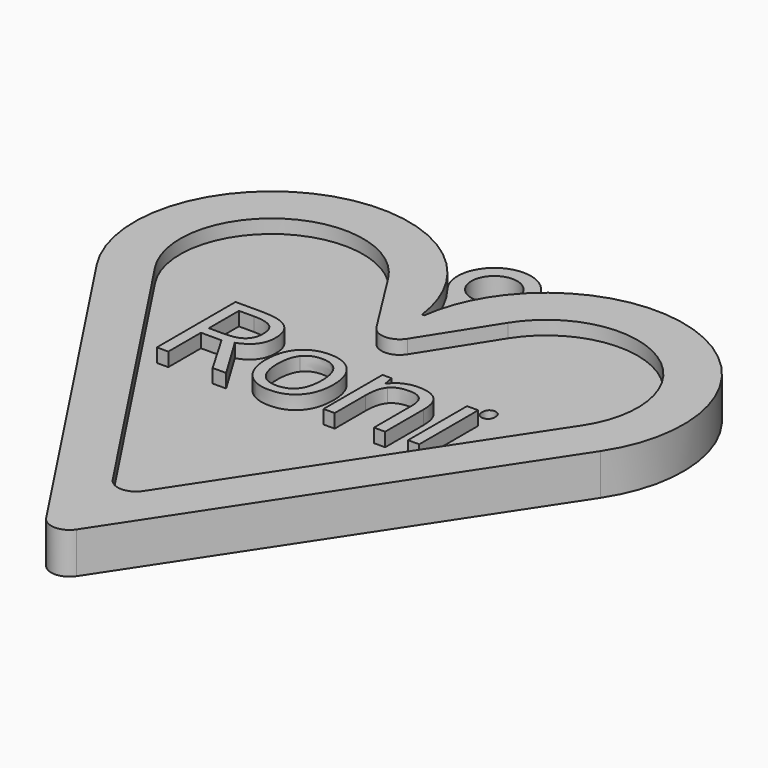
from build123d import *

# Parameters (mm, degrees)
F0_W     = 1.2206887795
F0_H     = 8.0556051444
F0_R     = 2.5
F1_DEPTH = 3
F2_DEPTH = 4.5
F3_R     = 2


# Not quite as in the source:
# - a feature names something its author has since deleted; it is built from what else it names


with BuildPart() as f1:
    # F0 (on Top) → F1 (new body)
    with BuildSketch(Plane.XY):
        with BuildLine():
            Line((-36.7494719235, 22.4924636665), (-36.8790277196, 22.5606875716))
            ThreePointArc((-36.8790277196, 22.5606875716), (-37.9113762546, 26.3820166599), (-39.9073666892, 29.800250368))
            ThreePointArc((-39.9073666892, 29.800250368), (-60.4879285093, 32.7852591337), (-64.2724077033, 12.336603447))
            Line((-64.2724077033, 12.336603447), (-36.7494719235, -29.406515819))
            Line((-36.7494719235, -29.406515819), (-9.2265361436, 12.336603447))
            ThreePointArc((-9.2265361436, 12.336603447), (-13.0110153192, 32.7852591205), (-33.5915771299, 29.8002504037))
            ThreePointArc((-33.5915771299, 29.8002504037), (-35.5875675836, 26.3820166807), (-36.6199161273, 22.5606875716))
            Line((-36.6199161273, 22.5606875716), (-36.7494719235, 22.4924636665))
        make_face()
        with BuildLine():
            Line((-36.7494719235, -20.3231824857), (-60.0980957767, 15.088897025))
            ThreePointArc((-60.0980957767, 15.088897025), (-57.1762344668, 28.9929037025), (-43.2999821807, 25.9419534093))
            Line((-43.2999821807, 25.9419534093), (-36.7494719235, 15.593484181))
            Line((-36.7494719235, 15.593484181), (-30.1989616662, 25.9419534093))
            ThreePointArc((-30.1989616662, 25.9419534093), (-16.3227093801, 28.9929037025), (-13.4008480702, 15.088897025))
            Line((-13.4008480702, 15.088897025), (-36.7494719235, -20.3231824857))
        make_face(mode=Mode.SUBTRACT)
        with BuildLine():
            ThreePointArc((-43.2999821807, 25.9419534093), (-57.1762344668, 28.9929037025), (-60.0980957767, 15.088897025))
            Line((-60.0980957767, 15.088897025), (-36.7494719235, -20.3231824857))
            Line((-36.7494719235, -20.3231824857), (-13.4008480702, 15.088897025))
            ThreePointArc((-13.4008480702, 15.088897025), (-16.3227093801, 28.9929037025), (-30.1989616662, 25.9419534093))
            Line((-30.1989616662, 25.9419534093), (-36.7494719235, 15.593484181))
            Line((-36.7494719235, 15.593484181), (-43.2999821807, 25.9419534093))
        make_face()
        with BuildLine():
            Line((-47.2641347396, 8.1347208725), (-49.5079441725, 8.1347208725))
            Line((-49.5079441725, 8.1347208725), (-49.5079441725, 3.6659180187))
            Line((-49.5079441725, 3.6659180187), (-50.7568569701, 3.6659180187))
            Line((-50.7568569701, 3.6659180187), (-50.7568569701, 14.4122128813))
            Line((-50.7568569701, 14.4122128813), (-47.8097990881, 14.4122128813))
            add(Edge.make_bspline(
                [(-47.8097990881, 14.4122128813), (-45.8317658249, 14.4122128813), (-44.8874372219, 13.6548683977)],
                knots=[0, 0, 0, 1, 1, 1], degree=2))
            add(Edge.make_bspline(
                [(-44.8874372219, 13.6548683977), (-43.9431086188, 12.897523914), (-43.9431086188, 11.3757789422)],
                knots=[0, 0, 0, 1, 1, 1], degree=2))
            add(Edge.make_bspline(
                [(-43.9431086188, 11.3757789422), (-43.9431086188, 9.2448655814), (-46.1045979991, 8.4945771023)],
                knots=[0, 0, 0, 1, 1, 1], degree=2))
            Line((-46.1045979991, 8.4945771023), (-43.1857641352, 3.6659180187))
            Line((-43.1857641352, 3.6659180187), (-44.6628210784, 3.6659180187))
            Line((-44.6628210784, 3.6659180187), (-47.2641347396, 8.1347208725))
        make_face(mode=Mode.SUBTRACT)
        with BuildLine():
            add(Edge.make_bspline(
                [(-35.6793513415, 10.7442665389), (-34.6832787054, 9.6188338202), (-34.6832787054, 7.7019525961)],
                knots=[0, 0, 0, 1, 1, 1], degree=2))
            add(Edge.make_bspline(
                [(-34.6832787054, 7.7019525961), (-34.6832787054, 5.7309753374), (-35.6746473385, 4.6243586307)],
                knots=[0, 0, 0, 1, 1, 1], degree=2))
            add(Edge.make_bspline(
                [(-35.6746473385, 4.6243586307), (-36.6660159716, 3.517741924), (-38.4159050891, 3.517741924)],
                knots=[0, 0, 0, 1, 1, 1], degree=2))
            add(Edge.make_bspline(
                [(-38.4159050891, 3.517741924), (-39.49782578, 3.517741924), (-40.3351383147, 4.0257742485)],
                knots=[0, 0, 0, 1, 1, 1], degree=2))
            add(Edge.make_bspline(
                [(-40.3351383147, 4.0257742485), (-41.1724508494, 4.5338065729), (-41.6287391408, 5.4816631782)],
                knots=[0, 0, 0, 1, 1, 1], degree=2))
            add(Edge.make_bspline(
                [(-41.6287391408, 5.4816631782), (-42.0850274322, 6.4295197835), (-42.0850274322, 7.7019525961)],
                knots=[0, 0, 0, 1, 1, 1], degree=2))
            add(Edge.make_bspline(
                [(-42.0850274322, 7.7019525961), (-42.0850274322, 9.6705778533), (-41.0995388029, 10.7701385555)],
                knots=[0, 0, 0, 1, 1, 1], degree=2))
            add(Edge.make_bspline(
                [(-41.0995388029, 10.7701385555), (-40.1140501735, 11.8696992577), (-38.3641610561, 11.8696992577)],
                knots=[0, 0, 0, 1, 1, 1], degree=2))
            add(Edge.make_bspline(
                [(-38.3641610561, 11.8696992577), (-36.6754239776, 11.8696992577), (-35.6793513415, 10.7442665389)],
                knots=[0, 0, 0, 1, 1, 1], degree=2))
        make_face(mode=Mode.SUBTRACT)
        with BuildLine():
            Line((-25.8091770384, 3.6659180187), (-27.0298658179, 3.6659180187))
            Line((-27.0298658179, 3.6659180187), (-27.0298658179, 8.8779533471))
            add(Edge.make_bspline(
                [(-27.0298658179, 8.8779533471), (-27.0298658179, 9.8610899749), (-27.477922104, 10.3467782851)],
                knots=[0, 0, 0, 1, 1, 1], degree=2))
            add(Edge.make_bspline(
                [(-27.477922104, 10.3467782851), (-27.9259783902, 10.8324665953), (-28.8832430015, 10.8324665953)],
                knots=[0, 0, 0, 1, 1, 1], degree=2))
            add(Edge.make_bspline(
                [(-28.8832430015, 10.8324665953), (-30.146267808, 10.8324665953), (-30.7342681836, 10.1492101589)],
                knots=[0, 0, 0, 1, 1, 1], degree=2))
            add(Edge.make_bspline(
                [(-30.7342681836, 10.1492101589), (-31.3222685591, 9.4659537226), (-31.3222685591, 7.8924647178)],
                knots=[0, 0, 0, 1, 1, 1], degree=2))
            Line((-31.3222685591, 7.8924647178), (-31.3222685591, 3.6659180187))
            Line((-31.3222685591, 3.6659180187), (-32.5429573386, 3.6659180187))
            Line((-32.5429573386, 3.6659180187), (-32.5429573386, 11.721523163))
            Line((-32.5429573386, 11.721523163), (-31.5504127047, 11.721523163))
            Line((-31.5504127047, 11.721523163), (-31.3528445786, 10.6184344586))
            Line((-31.3528445786, 10.6184344586), (-31.294044541, 10.6184344586))
            add(Edge.make_bspline(
                [(-31.294044541, 10.6184344586), (-30.9177243007, 11.2134908386), (-30.2415238689, 11.5415950481)],
                knots=[0, 0, 0, 1, 1, 1], degree=2))
            add(Edge.make_bspline(
                [(-30.2415238689, 11.5415950481), (-29.5653234371, 11.8696992577), (-28.7350669068, 11.8696992577)],
                knots=[0, 0, 0, 1, 1, 1], degree=2))
            add(Edge.make_bspline(
                [(-28.7350669068, 11.8696992577), (-27.2791779771, 11.8696992577), (-26.5441775077, 11.1676268093)],
                knots=[0, 0, 0, 1, 1, 1], degree=2))
            add(Edge.make_bspline(
                [(-26.5441775077, 11.1676268093), (-25.8091770384, 10.465554361), (-25.8091770384, 8.9202893741)],
                knots=[0, 0, 0, 1, 1, 1], degree=2))
            Line((-25.8091770384, 8.9202893741), (-25.8091770384, 3.6659180187))
        make_face(mode=Mode.SUBTRACT)
        with Locations((-22.693951049, 7.6937205909)):
            Rectangle(F0_W, F0_H, mode=Mode.SUBTRACT)
        with BuildLine():
            add(Edge.make_bspline(
                [(-23.2019833734, 13.2903081649), (-23.4077835048, 13.492580294), (-23.4077835048, 13.9041805569)],
                knots=[0, 0, 0, 1, 1, 1], degree=2))
            add(Edge.make_bspline(
                [(-23.4077835048, 13.9041805569), (-23.4077835048, 14.3228368242), (-23.2019833734, 14.5180529489)],
                knots=[0, 0, 0, 1, 1, 1], degree=2))
            add(Edge.make_bspline(
                [(-23.2019833734, 14.5180529489), (-22.996183242, 14.7132690736), (-22.6857190437, 14.7132690736)],
                knots=[0, 0, 0, 1, 1, 1], degree=2))
            add(Edge.make_bspline(
                [(-22.6857190437, 14.7132690736), (-22.3917188559, 14.7132690736), (-22.17886272, 14.5145249467)],
                knots=[0, 0, 0, 1, 1, 1], degree=2))
            add(Edge.make_bspline(
                [(-22.17886272, 14.5145249467), (-21.9660065841, 14.3157808197), (-21.9660065841, 13.9041805569)],
                knots=[0, 0, 0, 1, 1, 1], degree=2))
            add(Edge.make_bspline(
                [(-21.9660065841, 13.9041805569), (-21.9660065841, 13.492580294), (-22.17886272, 13.2903081649)],
                knots=[0, 0, 0, 1, 1, 1], degree=2))
            add(Edge.make_bspline(
                [(-22.17886272, 13.2903081649), (-22.3917188559, 13.0880360357), (-22.6857190437, 13.0880360357)],
                knots=[0, 0, 0, 1, 1, 1], degree=2))
            add(Edge.make_bspline(
                [(-22.6857190437, 13.0880360357), (-22.996183242, 13.0880360357), (-23.2019833734, 13.2903081649)],
                knots=[0, 0, 0, 1, 1, 1], degree=2))
        make_face(mode=Mode.SUBTRACT)
        with BuildLine():
            Line((-49.5079441725, 3.6659180187), (-49.5079441725, 8.1347208725))
            Line((-49.5079441725, 8.1347208725), (-47.2641347396, 8.1347208725))
            Line((-47.2641347396, 8.1347208725), (-44.6628210784, 3.6659180187))
            Line((-44.6628210784, 3.6659180187), (-43.1857641352, 3.6659180187))
            Line((-43.1857641352, 3.6659180187), (-46.1045979991, 8.4945771023))
            add(Edge.make_bspline(
                [(-43.9431086188, 11.3757789422), (-43.9431086188, 9.2448655814), (-46.1045979991, 8.4945771023)],
                knots=[0, 0, 0, 1, 1, 1], degree=2))
            add(Edge.make_bspline(
                [(-44.8874372219, 13.6548683977), (-43.9431086188, 12.897523914), (-43.9431086188, 11.3757789422)],
                knots=[0, 0, 0, 1, 1, 1], degree=2))
            add(Edge.make_bspline(
                [(-47.8097990881, 14.4122128813), (-45.8317658249, 14.4122128813), (-44.8874372219, 13.6548683977)],
                knots=[0, 0, 0, 1, 1, 1], degree=2))
            Line((-47.8097990881, 14.4122128813), (-50.7568569701, 14.4122128813))
            Line((-50.7568569701, 14.4122128813), (-50.7568569701, 3.6659180187))
            Line((-50.7568569701, 3.6659180187), (-49.5079441725, 3.6659180187))
        make_face()
        with BuildLine():
            Line((-47.7933350776, 9.2072335574), (-49.5079441725, 9.2072335574))
            Line((-49.5079441725, 9.2072335574), (-49.5079441725, 13.3161801814))
            Line((-49.5079441725, 13.3161801814), (-47.8827111347, 13.3161801814))
            add(Edge.make_bspline(
                [(-45.8646938459, 12.845779881), (-46.492678247, 13.3161801814), (-47.8827111347, 13.3161801814)],
                knots=[0, 0, 0, 1, 1, 1], degree=2))
            add(Edge.make_bspline(
                [(-45.2367094449, 11.3099229002), (-45.2367094449, 12.3753795806), (-45.8646938459, 12.845779881)],
                knots=[0, 0, 0, 1, 1, 1], degree=2))
            add(Edge.make_bspline(
                [(-45.8541098392, 9.7329058931), (-45.2367094449, 10.2585782288), (-45.2367094449, 11.3099229002)],
                knots=[0, 0, 0, 1, 1, 1], degree=2))
            add(Edge.make_bspline(
                [(-47.7933350776, 9.2072335574), (-46.4715102335, 9.2072335574), (-45.8541098392, 9.7329058931)],
                knots=[0, 0, 0, 1, 1, 1], degree=2))
        make_face(mode=Mode.SUBTRACT)
        with BuildLine():
            add(Edge.make_bspline(
                [(-34.6832787054, 7.7019525961), (-34.6832787054, 5.7309753374), (-35.6746473385, 4.6243586307)],
                knots=[0, 0, 0, 1, 1, 1], degree=2))
            add(Edge.make_bspline(
                [(-35.6793513415, 10.7442665389), (-34.6832787054, 9.6188338202), (-34.6832787054, 7.7019525961)],
                knots=[0, 0, 0, 1, 1, 1], degree=2))
            add(Edge.make_bspline(
                [(-38.3641610561, 11.8696992577), (-36.6754239776, 11.8696992577), (-35.6793513415, 10.7442665389)],
                knots=[0, 0, 0, 1, 1, 1], degree=2))
            add(Edge.make_bspline(
                [(-41.0995388029, 10.7701385555), (-40.1140501735, 11.8696992577), (-38.3641610561, 11.8696992577)],
                knots=[0, 0, 0, 1, 1, 1], degree=2))
            add(Edge.make_bspline(
                [(-42.0850274322, 7.7019525961), (-42.0850274322, 9.6705778533), (-41.0995388029, 10.7701385555)],
                knots=[0, 0, 0, 1, 1, 1], degree=2))
            add(Edge.make_bspline(
                [(-41.6287391408, 5.4816631782), (-42.0850274322, 6.4295197835), (-42.0850274322, 7.7019525961)],
                knots=[0, 0, 0, 1, 1, 1], degree=2))
            add(Edge.make_bspline(
                [(-40.3351383147, 4.0257742485), (-41.1724508494, 4.5338065729), (-41.6287391408, 5.4816631782)],
                knots=[0, 0, 0, 1, 1, 1], degree=2))
            add(Edge.make_bspline(
                [(-38.4159050891, 3.517741924), (-39.49782578, 3.517741924), (-40.3351383147, 4.0257742485)],
                knots=[0, 0, 0, 1, 1, 1], degree=2))
            add(Edge.make_bspline(
                [(-35.6746473385, 4.6243586307), (-36.6660159716, 3.517741924), (-38.4159050891, 3.517741924)],
                knots=[0, 0, 0, 1, 1, 1], degree=2))
        make_face()
        with BuildLine():
            add(Edge.make_bspline(
                [(-40.8196506241, 7.7019525961), (-40.8196506241, 6.1566876093), (-40.2022502299, 5.3487750934)],
                knots=[0, 0, 0, 1, 1, 1], degree=2))
            add(Edge.make_bspline(
                [(-40.2093062344, 10.0457220929), (-40.8196506241, 9.2589775904), (-40.8196506241, 7.7019525961)],
                knots=[0, 0, 0, 1, 1, 1], degree=2))
            add(Edge.make_bspline(
                [(-38.4017930801, 10.8324665953), (-39.5989618446, 10.8324665953), (-40.2093062344, 10.0457220929)],
                knots=[0, 0, 0, 1, 1, 1], degree=2))
            add(Edge.make_bspline(
                [(-36.5672319085, 10.0351380861), (-37.188160305, 10.8324665953), (-38.4017930801, 10.8324665953)],
                knots=[0, 0, 0, 1, 1, 1], degree=2))
            add(Edge.make_bspline(
                [(-35.946303512, 7.7019525961), (-35.946303512, 9.2378095769), (-36.5672319085, 10.0351380861)],
                knots=[0, 0, 0, 1, 1, 1], degree=2))
            add(Edge.make_bspline(
                [(-36.5672319085, 5.3452470911), (-35.946303512, 6.1496316048), (-35.946303512, 7.7019525961)],
                knots=[0, 0, 0, 1, 1, 1], degree=2))
            add(Edge.make_bspline(
                [(-38.3876810711, 4.5408625774), (-37.188160305, 4.5408625774), (-36.5672319085, 5.3452470911)],
                knots=[0, 0, 0, 1, 1, 1], degree=2))
            add(Edge.make_bspline(
                [(-40.2022502299, 5.3487750934), (-39.5848498356, 4.5408625774), (-38.3876810711, 4.5408625774)],
                knots=[0, 0, 0, 1, 1, 1], degree=2))
        make_face(mode=Mode.SUBTRACT)
        with BuildLine():
            ThreePointArc((-32.7494719235, 32.2553879707), (-38.0472432702, 36.03900919), (-39.9073666892, 29.800250368))
            ThreePointArc((-39.9073666892, 29.800250368), (-36.7494719008, 28.2553879707), (-33.5915771299, 29.8002504037))
            ThreePointArc((-33.5915771299, 29.8002504037), (-32.9658506968, 30.9576166453), (-32.7494719235, 32.2553879707))
        make_face()
        with Locations((-36.7494719235, 32.2553879707)):
            Circle(F0_R, mode=Mode.SUBTRACT)
        with BuildLine():
            add(Edge.make_bspline(
                [(-40.2093062344, 10.0457220929), (-40.8196506241, 9.2589775904), (-40.8196506241, 7.7019525961)],
                knots=[0, 0, 0, 1, 1, 1], degree=2))
            add(Edge.make_bspline(
                [(-40.8196506241, 7.7019525961), (-40.8196506241, 6.1566876093), (-40.2022502299, 5.3487750934)],
                knots=[0, 0, 0, 1, 1, 1], degree=2))
            add(Edge.make_bspline(
                [(-40.2022502299, 5.3487750934), (-39.5848498356, 4.5408625774), (-38.3876810711, 4.5408625774)],
                knots=[0, 0, 0, 1, 1, 1], degree=2))
            add(Edge.make_bspline(
                [(-38.3876810711, 4.5408625774), (-37.188160305, 4.5408625774), (-36.5672319085, 5.3452470911)],
                knots=[0, 0, 0, 1, 1, 1], degree=2))
            add(Edge.make_bspline(
                [(-36.5672319085, 5.3452470911), (-35.946303512, 6.1496316048), (-35.946303512, 7.7019525961)],
                knots=[0, 0, 0, 1, 1, 1], degree=2))
            add(Edge.make_bspline(
                [(-35.946303512, 7.7019525961), (-35.946303512, 9.2378095769), (-36.5672319085, 10.0351380861)],
                knots=[0, 0, 0, 1, 1, 1], degree=2))
            add(Edge.make_bspline(
                [(-36.5672319085, 10.0351380861), (-37.188160305, 10.8324665953), (-38.4017930801, 10.8324665953)],
                knots=[0, 0, 0, 1, 1, 1], degree=2))
            add(Edge.make_bspline(
                [(-38.4017930801, 10.8324665953), (-39.5989618446, 10.8324665953), (-40.2093062344, 10.0457220929)],
                knots=[0, 0, 0, 1, 1, 1], degree=2))
        make_face()
        with BuildLine():
            Line((-27.0298658179, 8.8779533471), (-27.0298658179, 3.6659180187))
            Line((-27.0298658179, 3.6659180187), (-25.8091770384, 3.6659180187))
            Line((-25.8091770384, 3.6659180187), (-25.8091770384, 8.9202893741))
            add(Edge.make_bspline(
                [(-26.5441775077, 11.1676268093), (-25.8091770384, 10.465554361), (-25.8091770384, 8.9202893741)],
                knots=[0, 0, 0, 1, 1, 1], degree=2))
            add(Edge.make_bspline(
                [(-28.7350669068, 11.8696992577), (-27.2791779771, 11.8696992577), (-26.5441775077, 11.1676268093)],
                knots=[0, 0, 0, 1, 1, 1], degree=2))
            add(Edge.make_bspline(
                [(-30.2415238689, 11.5415950481), (-29.5653234371, 11.8696992577), (-28.7350669068, 11.8696992577)],
                knots=[0, 0, 0, 1, 1, 1], degree=2))
            add(Edge.make_bspline(
                [(-31.294044541, 10.6184344586), (-30.9177243007, 11.2134908386), (-30.2415238689, 11.5415950481)],
                knots=[0, 0, 0, 1, 1, 1], degree=2))
            Line((-31.294044541, 10.6184344586), (-31.3528445786, 10.6184344586))
            Line((-31.3528445786, 10.6184344586), (-31.5504127047, 11.721523163))
            Line((-31.5504127047, 11.721523163), (-32.5429573386, 11.721523163))
            Line((-32.5429573386, 11.721523163), (-32.5429573386, 3.6659180187))
            Line((-32.5429573386, 3.6659180187), (-31.3222685591, 3.6659180187))
            Line((-31.3222685591, 3.6659180187), (-31.3222685591, 7.8924647178))
            add(Edge.make_bspline(
                [(-30.7342681836, 10.1492101589), (-31.3222685591, 9.4659537226), (-31.3222685591, 7.8924647178)],
                knots=[0, 0, 0, 1, 1, 1], degree=2))
            add(Edge.make_bspline(
                [(-28.8832430015, 10.8324665953), (-30.146267808, 10.8324665953), (-30.7342681836, 10.1492101589)],
                knots=[0, 0, 0, 1, 1, 1], degree=2))
            add(Edge.make_bspline(
                [(-27.477922104, 10.3467782851), (-27.9259783902, 10.8324665953), (-28.8832430015, 10.8324665953)],
                knots=[0, 0, 0, 1, 1, 1], degree=2))
            add(Edge.make_bspline(
                [(-27.0298658179, 8.8779533471), (-27.0298658179, 9.8610899749), (-27.477922104, 10.3467782851)],
                knots=[0, 0, 0, 1, 1, 1], degree=2))
        make_face()
        with BuildLine():
            Line((-49.5079441725, 13.3161801814), (-49.5079441725, 9.2072335574))
            Line((-49.5079441725, 9.2072335574), (-47.7933350776, 9.2072335574))
            add(Edge.make_bspline(
                [(-47.7933350776, 9.2072335574), (-46.4715102335, 9.2072335574), (-45.8541098392, 9.7329058931)],
                knots=[0, 0, 0, 1, 1, 1], degree=2))
            add(Edge.make_bspline(
                [(-45.8541098392, 9.7329058931), (-45.2367094449, 10.2585782288), (-45.2367094449, 11.3099229002)],
                knots=[0, 0, 0, 1, 1, 1], degree=2))
            add(Edge.make_bspline(
                [(-45.2367094449, 11.3099229002), (-45.2367094449, 12.3753795806), (-45.8646938459, 12.845779881)],
                knots=[0, 0, 0, 1, 1, 1], degree=2))
            add(Edge.make_bspline(
                [(-45.8646938459, 12.845779881), (-46.492678247, 13.3161801814), (-47.8827111347, 13.3161801814)],
                knots=[0, 0, 0, 1, 1, 1], degree=2))
            Line((-47.8827111347, 13.3161801814), (-49.5079441725, 13.3161801814))
        make_face()
        with BuildLine():
            ThreePointArc((-39.9073666892, 29.800250368), (-37.9113762546, 26.3820166599), (-36.8790277196, 22.5606875716))
            Line((-36.8790277196, 22.5606875716), (-36.7494719235, 22.4924636665))
            Line((-36.7494719235, 22.4924636665), (-36.6199161273, 22.5606875716))
            ThreePointArc((-36.6199161273, 22.5606875716), (-35.5875675836, 26.3820166807), (-33.5915771299, 29.8002504037))
            ThreePointArc((-33.5915771299, 29.8002504037), (-36.7494719008, 28.2553879707), (-39.9073666892, 29.800250368))
        make_face()
        with Locations((-22.693951049, 7.6937205909)):
            Rectangle(F0_W, F0_H)
    extrude(amount=F1_DEPTH)

    # F0 (on Top) → F2 (join)
    with BuildSketch(Plane.XY):
        with BuildLine():
            Line((-36.7494719235, 22.4924636665), (-36.8790277196, 22.5606875716))
            ThreePointArc((-36.8790277196, 22.5606875716), (-37.9113762546, 26.3820166599), (-39.9073666892, 29.800250368))
            ThreePointArc((-39.9073666892, 29.800250368), (-60.4879285093, 32.7852591337), (-64.2724077033, 12.336603447))
            Line((-64.2724077033, 12.336603447), (-36.7494719235, -29.406515819))
            Line((-36.7494719235, -29.406515819), (-9.2265361436, 12.336603447))
            ThreePointArc((-9.2265361436, 12.336603447), (-13.0110153192, 32.7852591205), (-33.5915771299, 29.8002504037))
            ThreePointArc((-33.5915771299, 29.8002504037), (-35.5875675836, 26.3820166807), (-36.6199161273, 22.5606875716))
            Line((-36.6199161273, 22.5606875716), (-36.7494719235, 22.4924636665))
        make_face()
        with BuildLine():
            Line((-36.7494719235, -20.3231824857), (-60.0980957767, 15.088897025))
            ThreePointArc((-60.0980957767, 15.088897025), (-57.1762344668, 28.9929037025), (-43.2999821807, 25.9419534093))
            Line((-43.2999821807, 25.9419534093), (-36.7494719235, 15.593484181))
            Line((-36.7494719235, 15.593484181), (-30.1989616662, 25.9419534093))
            ThreePointArc((-30.1989616662, 25.9419534093), (-16.3227093801, 28.9929037025), (-13.4008480702, 15.088897025))
            Line((-13.4008480702, 15.088897025), (-36.7494719235, -20.3231824857))
        make_face(mode=Mode.SUBTRACT)
        with BuildLine():
            add(Edge.make_bspline(
                [(-34.6832787054, 7.7019525961), (-34.6832787054, 5.7309753374), (-35.6746473385, 4.6243586307)],
                knots=[0, 0, 0, 1, 1, 1], degree=2))
            add(Edge.make_bspline(
                [(-35.6793513415, 10.7442665389), (-34.6832787054, 9.6188338202), (-34.6832787054, 7.7019525961)],
                knots=[0, 0, 0, 1, 1, 1], degree=2))
            add(Edge.make_bspline(
                [(-38.3641610561, 11.8696992577), (-36.6754239776, 11.8696992577), (-35.6793513415, 10.7442665389)],
                knots=[0, 0, 0, 1, 1, 1], degree=2))
            add(Edge.make_bspline(
                [(-41.0995388029, 10.7701385555), (-40.1140501735, 11.8696992577), (-38.3641610561, 11.8696992577)],
                knots=[0, 0, 0, 1, 1, 1], degree=2))
            add(Edge.make_bspline(
                [(-42.0850274322, 7.7019525961), (-42.0850274322, 9.6705778533), (-41.0995388029, 10.7701385555)],
                knots=[0, 0, 0, 1, 1, 1], degree=2))
            add(Edge.make_bspline(
                [(-41.6287391408, 5.4816631782), (-42.0850274322, 6.4295197835), (-42.0850274322, 7.7019525961)],
                knots=[0, 0, 0, 1, 1, 1], degree=2))
            add(Edge.make_bspline(
                [(-40.3351383147, 4.0257742485), (-41.1724508494, 4.5338065729), (-41.6287391408, 5.4816631782)],
                knots=[0, 0, 0, 1, 1, 1], degree=2))
            add(Edge.make_bspline(
                [(-38.4159050891, 3.517741924), (-39.49782578, 3.517741924), (-40.3351383147, 4.0257742485)],
                knots=[0, 0, 0, 1, 1, 1], degree=2))
            add(Edge.make_bspline(
                [(-35.6746473385, 4.6243586307), (-36.6660159716, 3.517741924), (-38.4159050891, 3.517741924)],
                knots=[0, 0, 0, 1, 1, 1], degree=2))
        make_face()
        with BuildLine():
            add(Edge.make_bspline(
                [(-40.8196506241, 7.7019525961), (-40.8196506241, 6.1566876093), (-40.2022502299, 5.3487750934)],
                knots=[0, 0, 0, 1, 1, 1], degree=2))
            add(Edge.make_bspline(
                [(-40.2093062344, 10.0457220929), (-40.8196506241, 9.2589775904), (-40.8196506241, 7.7019525961)],
                knots=[0, 0, 0, 1, 1, 1], degree=2))
            add(Edge.make_bspline(
                [(-38.4017930801, 10.8324665953), (-39.5989618446, 10.8324665953), (-40.2093062344, 10.0457220929)],
                knots=[0, 0, 0, 1, 1, 1], degree=2))
            add(Edge.make_bspline(
                [(-36.5672319085, 10.0351380861), (-37.188160305, 10.8324665953), (-38.4017930801, 10.8324665953)],
                knots=[0, 0, 0, 1, 1, 1], degree=2))
            add(Edge.make_bspline(
                [(-35.946303512, 7.7019525961), (-35.946303512, 9.2378095769), (-36.5672319085, 10.0351380861)],
                knots=[0, 0, 0, 1, 1, 1], degree=2))
            add(Edge.make_bspline(
                [(-36.5672319085, 5.3452470911), (-35.946303512, 6.1496316048), (-35.946303512, 7.7019525961)],
                knots=[0, 0, 0, 1, 1, 1], degree=2))
            add(Edge.make_bspline(
                [(-38.3876810711, 4.5408625774), (-37.188160305, 4.5408625774), (-36.5672319085, 5.3452470911)],
                knots=[0, 0, 0, 1, 1, 1], degree=2))
            add(Edge.make_bspline(
                [(-40.2022502299, 5.3487750934), (-39.5848498356, 4.5408625774), (-38.3876810711, 4.5408625774)],
                knots=[0, 0, 0, 1, 1, 1], degree=2))
        make_face(mode=Mode.SUBTRACT)
        with BuildLine():
            Line((-27.0298658179, 8.8779533471), (-27.0298658179, 3.6659180187))
            Line((-27.0298658179, 3.6659180187), (-25.8091770384, 3.6659180187))
            Line((-25.8091770384, 3.6659180187), (-25.8091770384, 8.9202893741))
            add(Edge.make_bspline(
                [(-26.5441775077, 11.1676268093), (-25.8091770384, 10.465554361), (-25.8091770384, 8.9202893741)],
                knots=[0, 0, 0, 1, 1, 1], degree=2))
            add(Edge.make_bspline(
                [(-28.7350669068, 11.8696992577), (-27.2791779771, 11.8696992577), (-26.5441775077, 11.1676268093)],
                knots=[0, 0, 0, 1, 1, 1], degree=2))
            add(Edge.make_bspline(
                [(-30.2415238689, 11.5415950481), (-29.5653234371, 11.8696992577), (-28.7350669068, 11.8696992577)],
                knots=[0, 0, 0, 1, 1, 1], degree=2))
            add(Edge.make_bspline(
                [(-31.294044541, 10.6184344586), (-30.9177243007, 11.2134908386), (-30.2415238689, 11.5415950481)],
                knots=[0, 0, 0, 1, 1, 1], degree=2))
            Line((-31.294044541, 10.6184344586), (-31.3528445786, 10.6184344586))
            Line((-31.3528445786, 10.6184344586), (-31.5504127047, 11.721523163))
            Line((-31.5504127047, 11.721523163), (-32.5429573386, 11.721523163))
            Line((-32.5429573386, 11.721523163), (-32.5429573386, 3.6659180187))
            Line((-32.5429573386, 3.6659180187), (-31.3222685591, 3.6659180187))
            Line((-31.3222685591, 3.6659180187), (-31.3222685591, 7.8924647178))
            add(Edge.make_bspline(
                [(-30.7342681836, 10.1492101589), (-31.3222685591, 9.4659537226), (-31.3222685591, 7.8924647178)],
                knots=[0, 0, 0, 1, 1, 1], degree=2))
            add(Edge.make_bspline(
                [(-28.8832430015, 10.8324665953), (-30.146267808, 10.8324665953), (-30.7342681836, 10.1492101589)],
                knots=[0, 0, 0, 1, 1, 1], degree=2))
            add(Edge.make_bspline(
                [(-27.477922104, 10.3467782851), (-27.9259783902, 10.8324665953), (-28.8832430015, 10.8324665953)],
                knots=[0, 0, 0, 1, 1, 1], degree=2))
            add(Edge.make_bspline(
                [(-27.0298658179, 8.8779533471), (-27.0298658179, 9.8610899749), (-27.477922104, 10.3467782851)],
                knots=[0, 0, 0, 1, 1, 1], degree=2))
        make_face()
        with BuildLine():
            Line((-49.5079441725, 3.6659180187), (-49.5079441725, 8.1347208725))
            Line((-49.5079441725, 8.1347208725), (-47.2641347396, 8.1347208725))
            Line((-47.2641347396, 8.1347208725), (-44.6628210784, 3.6659180187))
            Line((-44.6628210784, 3.6659180187), (-43.1857641352, 3.6659180187))
            Line((-43.1857641352, 3.6659180187), (-46.1045979991, 8.4945771023))
            add(Edge.make_bspline(
                [(-43.9431086188, 11.3757789422), (-43.9431086188, 9.2448655814), (-46.1045979991, 8.4945771023)],
                knots=[0, 0, 0, 1, 1, 1], degree=2))
            add(Edge.make_bspline(
                [(-44.8874372219, 13.6548683977), (-43.9431086188, 12.897523914), (-43.9431086188, 11.3757789422)],
                knots=[0, 0, 0, 1, 1, 1], degree=2))
            add(Edge.make_bspline(
                [(-47.8097990881, 14.4122128813), (-45.8317658249, 14.4122128813), (-44.8874372219, 13.6548683977)],
                knots=[0, 0, 0, 1, 1, 1], degree=2))
            Line((-47.8097990881, 14.4122128813), (-50.7568569701, 14.4122128813))
            Line((-50.7568569701, 14.4122128813), (-50.7568569701, 3.6659180187))
            Line((-50.7568569701, 3.6659180187), (-49.5079441725, 3.6659180187))
        make_face()
        with BuildLine():
            Line((-47.7933350776, 9.2072335574), (-49.5079441725, 9.2072335574))
            Line((-49.5079441725, 9.2072335574), (-49.5079441725, 13.3161801814))
            Line((-49.5079441725, 13.3161801814), (-47.8827111347, 13.3161801814))
            add(Edge.make_bspline(
                [(-45.8646938459, 12.845779881), (-46.492678247, 13.3161801814), (-47.8827111347, 13.3161801814)],
                knots=[0, 0, 0, 1, 1, 1], degree=2))
            add(Edge.make_bspline(
                [(-45.2367094449, 11.3099229002), (-45.2367094449, 12.3753795806), (-45.8646938459, 12.845779881)],
                knots=[0, 0, 0, 1, 1, 1], degree=2))
            add(Edge.make_bspline(
                [(-45.8541098392, 9.7329058931), (-45.2367094449, 10.2585782288), (-45.2367094449, 11.3099229002)],
                knots=[0, 0, 0, 1, 1, 1], degree=2))
            add(Edge.make_bspline(
                [(-47.7933350776, 9.2072335574), (-46.4715102335, 9.2072335574), (-45.8541098392, 9.7329058931)],
                knots=[0, 0, 0, 1, 1, 1], degree=2))
        make_face(mode=Mode.SUBTRACT)
        with Locations((-22.693951049, 7.6937205909)):
            Rectangle(F0_W, F0_H)
    extrude(amount=F2_DEPTH)

    # F3
    f3_edges = [f1.edges().sort_by_distance(p)[0] for p in [
        (-36.749472, -29.406516, 2.25),
        (-36.749472, -20.323182, 3.75),
        (-36.749472, 15.593484, 3.75),
    ]]
    fillet(f3_edges, radius=F3_R)


solid = f1.part
